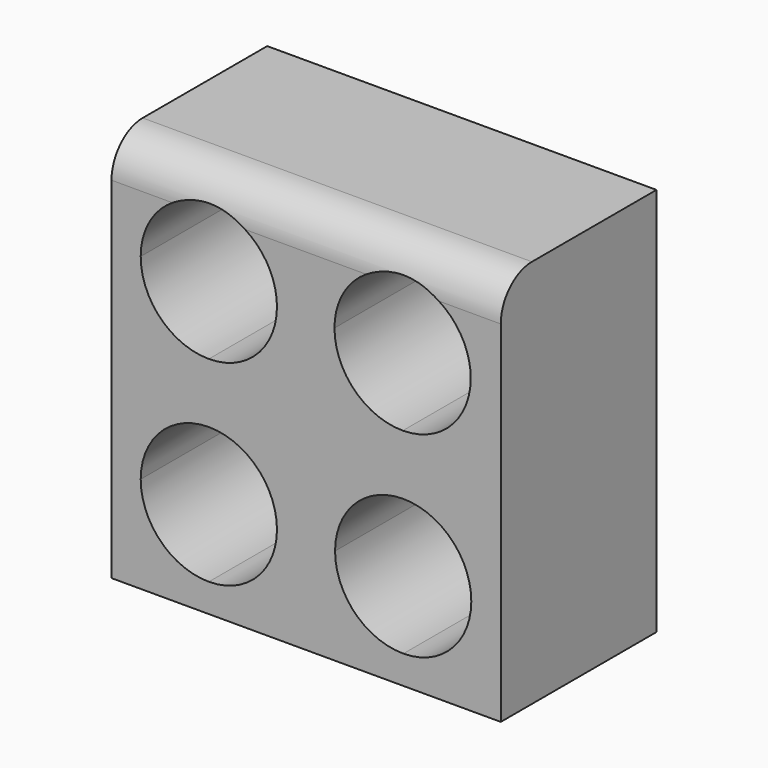
from build123d import *

# Parameters (mm, degrees)
F1_DEPTH    = 25.4
F2_T1_DEPTH = 76.2


# Not quite as in the source:
# - a fillet or chamfer that OpenCascade refuses, or shapes differently, is made with other operations: its cross-section is extruded or revolved along the edge and cut away or added


with BuildPart() as f1:
    # F0 (on Front) → F1 (new body)
    with BuildSketch(Plane.XZ):
        with BuildLine():
            Line((-12.7, 25.4), (-25.4, 25.4))
            Line((-25.4, 25.4), (-25.4, 12.798297219))
            Line((-25.4, 12.798297219), (-21.59, 12.798297219))
            ThreePointArc((-21.59, 12.798297219), (-18.9861792847, 19.0844765037), (-12.7, 21.688297219))
            Line((-12.7, 21.688297219), (-12.7, 25.4))
        make_face()
        with BuildLine():
            Line((0, 25.4), (-12.7, 25.4))
            Line((-12.7, 25.4), (-12.7, 21.688297219))
            ThreePointArc((-12.7, 21.688297219), (-6.4138207153, 19.0844765037), (-3.81, 12.798297219))
            Line((-3.81, 12.798297219), (0, 12.798297219))
            Line((0, 12.798297219), (0, 25.4))
        make_face()
        with BuildLine():
            Line((-21.59, 12.798297219), (-25.4, 12.798297219))
            Line((-25.4, 12.798297219), (-25.4, 0))
            Line((-25.4, 0), (-12.7, 0))
            Line((-12.7, 0), (-12.7, 3.908297219))
            ThreePointArc((-12.7, 3.908297219), (-18.9861792847, 6.5121179342), (-21.59, 12.798297219))
        make_face()
        with BuildLine():
            Line((12.5505886972, 25.4), (0, 25.4))
            Line((0, 25.4), (0, 12.798297219))
            Line((0, 12.798297219), (3.6976524143, 12.798297219))
            ThreePointArc((3.6976524143, 12.798297219), (6.2922356041, 19.0752253837), (12.5615055494, 21.6882587679))
            Line((12.5615055494, 21.6882587679), (12.5505886972, 25.4))
        make_face()
        with BuildLine():
            Line((-12.7, 0), (-25.4, 0))
            Line((-25.4, 0), (-25.4, -12.798297219))
            Line((-25.4, -12.798297219), (-21.59, -12.798297219))
            ThreePointArc((-21.59, -12.798297219), (-18.9861792847, -6.5121179342), (-12.7, -3.908297219))
            Line((-12.7, -3.908297219), (-12.7, 0))
        make_face()
        with BuildLine():
            Line((25.4, 25.4), (12.5505886972, 25.4))
            Line((12.5505886972, 25.4), (12.5615055494, 21.6882587679))
            ThreePointArc((12.5615055494, 21.6882587679), (18.8645805791, 19.0937140292), (21.4776524143, 12.798297219))
            Line((21.4776524143, 12.798297219), (25.4, 12.798297219))
            Line((25.4, 12.798297219), (25.4, 25.4))
        make_face()
        with BuildLine():
            Line((-21.59, -12.798297219), (-25.4, -12.798297219))
            Line((-25.4, -12.798297219), (-25.4, -25.4))
            Line((-25.4, -25.4), (-12.7, -25.4))
            Line((-12.7, -25.4), (-12.7, -21.688297219))
            ThreePointArc((-12.7, -21.688297219), (-18.9861792847, -19.0844765037), (-21.59, -12.798297219))
        make_face()
        with BuildLine():
            Line((25.4, 0), (25.4, 12.798297219))
            Line((25.4, 12.798297219), (21.4776524143, 12.798297219))
            ThreePointArc((21.4776524143, 12.798297219), (18.8830692245, 6.5213690542), (12.6137992792, 3.90833567))
            Line((12.6137992792, 3.90833567), (12.6252943486, 0))
            Line((12.6252943486, 0), (25.4, 0))
        make_face()
        with BuildLine():
            Line((3.7729362829, -12.798297219), (0, -12.798297219))
            Line((0, -12.798297219), (0, -25.4))
            Line((0, -25.4), (12.7, -25.4))
            Line((12.7, -25.4), (12.6890831478, -21.6882587679))
            ThreePointArc((12.6890831478, -21.6882587679), (6.3860081181, -19.0937140292), (3.7729362829, -12.798297219))
        make_face()
        with BuildLine():
            Line((0, -25.4), (0, -12.798297219))
            Line((0, -12.798297219), (-3.81, -12.798297219))
            ThreePointArc((-3.81, -12.798297219), (-6.4138207153, -19.0844765037), (-12.7, -21.688297219))
            Line((-12.7, -21.688297219), (-12.7, -25.4))
            Line((-12.7, -25.4), (0, -25.4))
        make_face()
        with BuildLine():
            Line((25.4, 0), (12.6252943486, 0))
            Line((12.6252943486, 0), (12.636789418, -3.90833567))
            ThreePointArc((12.636789418, -3.90833567), (18.9398644476, -6.5028804088), (21.5529362829, -12.798297219))
            Line((21.5529362829, -12.798297219), (25.4, -12.798297219))
            Line((25.4, -12.798297219), (25.4, 0))
        make_face()
        with BuildLine():
            Line((25.4, -25.4), (25.4, -12.798297219))
            Line((25.4, -12.798297219), (21.5529362829, -12.798297219))
            ThreePointArc((21.5529362829, -12.798297219), (18.9583530931, -19.0752253837), (12.6890831478, -21.6882587679))
            Line((12.6890831478, -21.6882587679), (12.7, -25.4))
            Line((12.7, -25.4), (25.4, -25.4))
        make_face()
        with BuildLine():
            Line((3.6976524143, 12.798297219), (0, 12.798297219))
            Line((0, 12.798297219), (0, 0))
            Line((0, 0), (12.6252943486, 0))
            Line((12.6252943486, 0), (12.6137992792, 3.90833567))
            ThreePointArc((12.6137992792, 3.90833567), (6.3107242496, 6.5028804088), (3.6976524143, 12.798297219))
        make_face()
        with BuildLine():
            Line((12.6252943486, 0), (0, 0))
            Line((0, 0), (0, -12.798297219))
            Line((0, -12.798297219), (3.7729362829, -12.798297219))
            ThreePointArc((3.7729362829, -12.798297219), (6.3675194726, -6.5213690542), (12.636789418, -3.90833567))
            Line((12.636789418, -3.90833567), (12.6252943486, 0))
        make_face()
        with BuildLine():
            Line((0, 0), (0, 12.798297219))
            Line((0, 12.798297219), (-3.81, 12.798297219))
            ThreePointArc((-3.81, 12.798297219), (-6.4138207153, 6.5121179342), (-12.7, 3.908297219))
            Line((-12.7, 3.908297219), (-12.7, 0))
            Line((-12.7, 0), (0, 0))
        make_face()
        with BuildLine():
            Line((0, 0), (-12.7, 0))
            Line((-12.7, 0), (-12.7, -3.908297219))
            ThreePointArc((-12.7, -3.908297219), (-6.4138207153, -6.5121179342), (-3.81, -12.798297219))
            Line((-3.81, -12.798297219), (0, -12.798297219))
            Line((0, -12.798297219), (0, 0))
        make_face()
    extrude(amount=F1_DEPTH)

    # F2: fillet of radius 5.08 on 1 edges, made by hand

    # F2_s2 → F2_t1 (cut)
    with BuildSketch(Plane.YZ.offset(-38.1)):
        with BuildLine():
            ThreePointArc((-20.32, 25.4), (-23.9121024484, 23.9121024484), (-25.4, 20.32))
            Line((-25.4, 20.32), (-25.4, 25.4))
            Line((-25.4, 25.4), (-20.32, 25.4))
        make_face()
    extrude(amount=F2_T1_DEPTH, mode=Mode.SUBTRACT)


solid = f1.part
